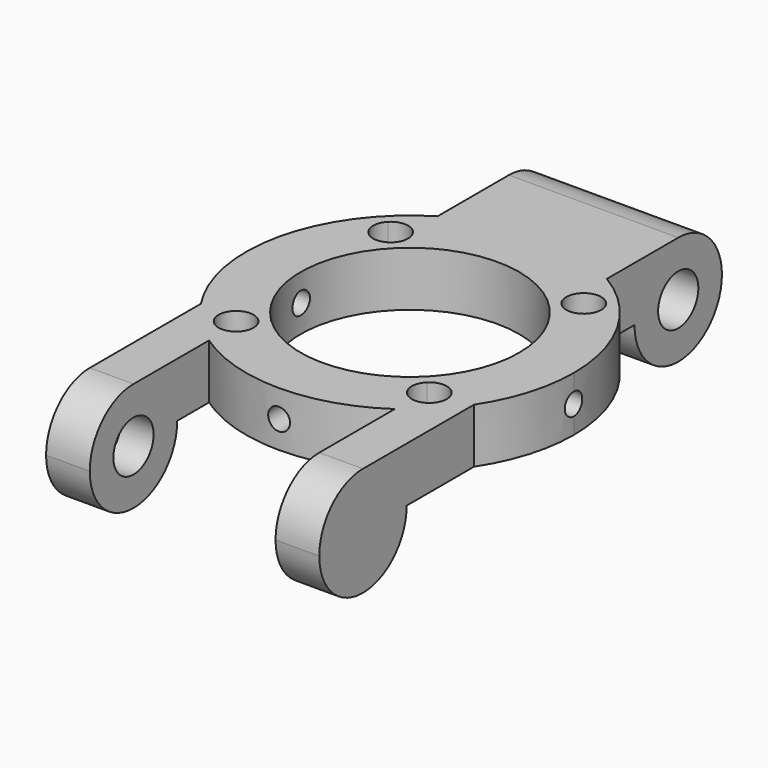
from build123d import *

# Parameters (mm, degrees)
F0_R      = 10
F1_DEPTH  = 5
F2_W      = 15.5
F2_H      = 10
F2_W_2    = 4
F3_DEPTH  = 5
F4_R      = 2.3
F5_DEPTH  = 22.751
F7_DEPTH  = 4
F8_R      = 2.3
F9_DEPTH  = 3
F10_R     = 2.3
F11_DEPTH = 3
F12_R     = 4.99999
F13_R     = 1
F14_DEPTH = 25
F15_R     = 1
F16_DEPTH = 25


# Not quite as in the source:
# - a fillet or chamfer is up to 0.001 mm smaller than in the source, because OpenCascade refuses the exact size


with BuildPart() as f1:
    # F0 (on Top) → F1 (new body)
    with BuildSketch(Plane.XY):
        with BuildLine():
            ThreePointArc((7.75, 12.842799539), (0, 15), (-7.75, 12.842799539))
            ThreePointArc((-7.75, 12.842799539), (-14.634921734, 3.289234841), (-12.5, -8.2915619759))
            ThreePointArc((-12.5, -8.2915619759), (-10.6951593818, -10.5172984077), (-8.5, -12.3592070943))
            ThreePointArc((-8.5, -12.3592070943), (0, -15), (8.5, -12.3592070943))
            ThreePointArc((8.5, -12.3592070943), (10.6951593818, -10.5172984077), (12.5, -8.2915619759))
            ThreePointArc((12.5, -8.2915619759), (14.3614066163, -4.3301270189), (15, 0))
            ThreePointArc((15, 0), (13.0623504776, 7.3739406019), (7.75, 12.842799539))
        make_face()
        Circle(F0_R, mode=Mode.SUBTRACT)
        with BuildLine():
            Line((-7.75, 26), (-7.75, 12.842799539))
            ThreePointArc((-7.75, 12.842799539), (0, 15), (7.75, 12.842799539))
            Line((7.75, 12.842799539), (7.75, 26))
            Line((7.75, 26), (-7.75, 26))
        make_face()
        with BuildLine():
            ThreePointArc((-8.5, -12.3592070943), (-10.6951593818, -10.5172984077), (-12.5, -8.2915619759))
            Line((-12.5, -8.2915619759), (-12.5, -26))
            Line((-12.5, -26), (-8.5, -26))
            Line((-8.5, -26), (-8.5, -12.3592070943))
        make_face()
        with BuildLine():
            ThreePointArc((12.5, -8.2915619759), (10.6951593818, -10.5172984077), (8.5, -12.3592070943))
            Line((8.5, -12.3592070943), (8.5, -26))
            Line((8.5, -26), (12.5, -26))
            Line((12.5, -26), (12.5, -8.2915619759))
        make_face()
    extrude(amount=F1_DEPTH)

    # F2 (on face) → F3 (join)
    with BuildSketch(Plane(origin=(0, 0, 0), x_dir=(1, 0, 0), z_dir=(0, 0, -1))):
        with Locations((0, -21)):
            Rectangle(F2_W, F2_H)
        with Locations((-10.5, 21)):
            Rectangle(F2_W_2, F2_H)
        with Locations((10.5, 21)):
            Rectangle(F2_W_2, F2_H)
    extrude(amount=F3_DEPTH)

    # F4 (on face) → F5 (cut, through all)
    with BuildSketch(Plane(origin=(-7.75, 0, 0), x_dir=(0, -1, 0), z_dir=(-1, 0, 0))):
        with Locations((-21, 0)):
            Circle(F4_R)
    extrude(amount=-F5_DEPTH, mode=Mode.SUBTRACT)

    # F6 (on face) → F7 (cut)
    with BuildSketch(Plane.XY.offset(5)):
        with BuildLine():
            ThreePointArc((10.4388347648, -8.8388347648), (9.4511282566, -7.3606275128), (7.7074639149, -7.7074639149))
            Line((7.7074639149, -7.7074639149), (9.9702056147, -9.9702056147))
            ThreePointArc((9.9702056147, -9.9702056147), (10.3170420168, -9.4511282566), (10.4388347648, -8.8388347648))
        make_face()
        with BuildLine():
            Line((9.9702056147, -9.9702056147), (7.7074639149, -7.7074639149))
            ThreePointArc((7.7074639149, -7.7074639149), (7.7074639149, -9.9702056147), (9.9702056147, -9.9702056147))
        make_face()
        with BuildLine():
            ThreePointArc((9.9702056147, 9.9702056147), (7.7074639149, 9.9702056147), (7.7074639149, 7.7074639149))
            Line((7.7074639149, 7.7074639149), (9.9702056147, 9.9702056147))
        make_face()
        with BuildLine():
            Line((9.9702056147, 9.9702056147), (7.7074639149, 7.7074639149))
            ThreePointArc((7.7074639149, 7.7074639149), (9.4511282566, 7.3606275128), (10.4388347648, 8.8388347648))
            ThreePointArc((10.4388347648, 8.8388347648), (10.3170420168, 9.4511282566), (9.9702056147, 9.9702056147))
        make_face()
        with BuildLine():
            ThreePointArc((-9.9702056147, 9.9702056147), (-9.9702056147, 7.7074639149), (-7.7074639149, 7.7074639149))
            Line((-7.7074639149, 7.7074639149), (-9.9702056147, 9.9702056147))
        make_face()
        with BuildLine():
            Line((-9.9702056147, 9.9702056147), (-7.7074639149, 7.7074639149))
            ThreePointArc((-7.7074639149, 7.7074639149), (-7.3606275128, 8.226541273), (-7.2388347648, 8.8388347648))
            ThreePointArc((-7.2388347648, 8.8388347648), (-8.226541273, 10.3170420168), (-9.9702056147, 9.9702056147))
        make_face()
        with BuildLine():
            ThreePointArc((-7.2388347648, -8.8388347648), (-7.3606275128, -8.226541273), (-7.7074639149, -7.7074639149))
            Line((-7.7074639149, -7.7074639149), (-9.9702056147, -9.9702056147))
            ThreePointArc((-9.9702056147, -9.9702056147), (-8.226541273, -10.3170420168), (-7.2388347648, -8.8388347648))
        make_face()
        with BuildLine():
            Line((-9.9702056147, -9.9702056147), (-7.7074639149, -7.7074639149))
            ThreePointArc((-7.7074639149, -7.7074639149), (-9.9702056147, -7.7074639149), (-9.9702056147, -9.9702056147))
        make_face()
    extrude(amount=-F7_DEPTH, mode=Mode.SUBTRACT)

    # F8 (on face) → F9 (cut)
    with BuildSketch(Plane.YZ.offset(-8.5)):
        with Locations((-21, 0)):
            Circle(F8_R)
    extrude(amount=-F9_DEPTH, mode=Mode.SUBTRACT)

    # F10 (on face) → F11 (cut)
    with BuildSketch(Plane(origin=(8.5, 0, 0), x_dir=(0, -1, 0), z_dir=(-1, 0, 0))):
        with Locations((21, 0)):
            Circle(F10_R)
    extrude(amount=-F11_DEPTH, mode=Mode.SUBTRACT)

    # F12 (radius 5 in the source; OpenCascade refuses exactly that, so slightly less here)
    f12_edges = [f1.edges().sort_by_distance(p)[0] for p in [
        (0, 26, -5),
        (0, 16, -5),
        (0, 26, 5),
        (-10.5, -26, -5),
        (-10.5, -26, 5),
        (10.5, -26, 5),
        (10.5, -26, -5),
        (-10.5, -16, -5),
        (10.5, -16, -5),
    ]]
    fillet(f12_edges, radius=F12_R)

    # F13 (on Right) → F14 (cut, symmetric)
    with BuildSketch(Plane.YZ):
        with Locations((0, 2.5)):
            Circle(F13_R)
    extrude(amount=F14_DEPTH, both=True, mode=Mode.SUBTRACT)

    # F15 (on Front) → F16 (cut)
    with BuildSketch(Plane.XZ):
        with Locations((0, 2.5)):
            Circle(F15_R)
    extrude(amount=F16_DEPTH, mode=Mode.SUBTRACT)


solid = f1.part
